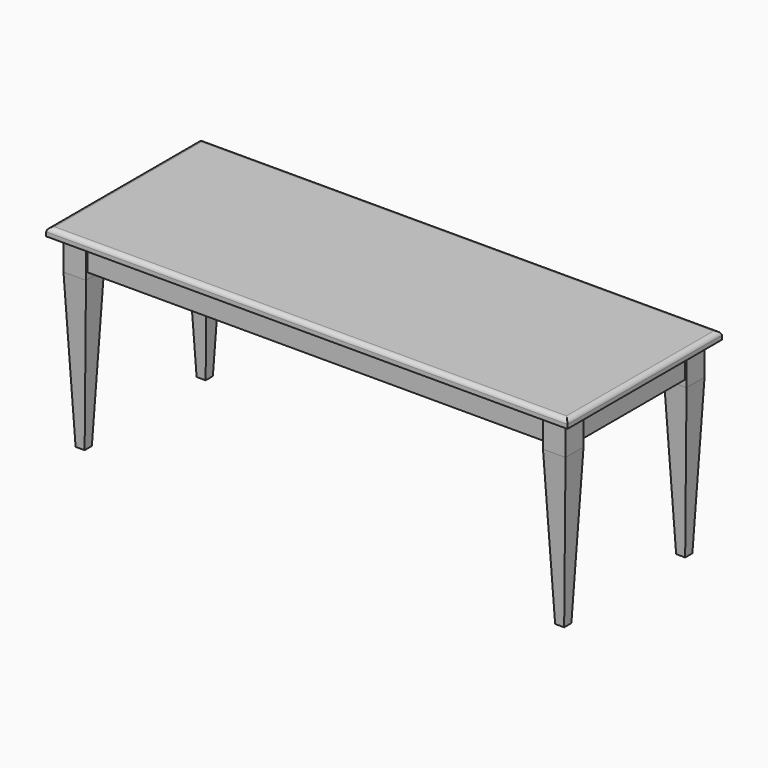
from build123d import *

# Parameters (mm, degrees)
F0_W        = 2057.4
F0_H        = 762
F1_DEPTH    = 15.875
F2_W        = 2057.4
F2_H        = 762
F3_DEPTH    = 15.875
F4_T1_DEPTH = 2151.3177665567
F4_T3_DEPTH = 855.9177665567
F6_W        = 88.9
F6_H        = 88.9
F7_DEPTH    = 127
F9_W        = 1968.5
F9_H        = 673.1
F10_DEPTH   = 101.6
F11_T       = -25.4
F12_W       = 88.9
F12_H       = 88.9
F13_DEPTH   = 609.6
F13_TAPER   = 2.5


# Not quite as in the source:
# - a fillet or chamfer that OpenCascade refuses, or shapes differently, is made with other operations: its cross-section is extruded or revolved along the edge and cut away or added


with BuildPart() as f1:
    # F0 (on Top) → F1 (new body)
    with BuildSketch(Plane.XY):
        Rectangle(F0_W, F0_H)
    extrude(amount=F1_DEPTH)

    # F6 (on face) → F7 (join)
    with BuildSketch(Plane(origin=(0, 0, 0), x_dir=(1, 0, 0), z_dir=(0, 0, -1))):
        with Locations((-946.15, 298.45)):
            Rectangle(F6_W, F6_H)
        with Locations((-946.15, -298.45)):
            Rectangle(F6_W, F6_H)
    extrude(amount=F7_DEPTH)

    # F8: F1 across plane


with BuildPart() as f3:
    # F2 (on face) → F3 (new body)
    with BuildSketch(Plane.XY.offset(15.875)):
        Rectangle(F2_W, F2_H)
    extrude(amount=F3_DEPTH)

    # F4: fillet of radius 19.05 on 4 edges, made by hand

    # F4_s2 → F4_t1 (cut)
    with BuildSketch(Plane.YZ.offset(-1075.6588832784)):
        with BuildLine():
            ThreePointArc((-381, 15.875), (-374.5131688129, 27.2496778315), (-362.2164466887, 31.75))
            Line((-362.2164466887, 31.75), (-381, 31.75))
            Line((-381, 31.75), (-381, 15.875))
        make_face()
        with BuildLine():
            ThreePointArc((381, 15.875), (374.5131688129, 27.2496778315), (362.2164466887, 31.75))
            Line((362.2164466887, 31.75), (381, 31.75))
            Line((381, 31.75), (381, 15.875))
        make_face()
    extrude(amount=F4_T1_DEPTH, mode=Mode.SUBTRACT)

    # F4_s4 → F4_t3 (cut)
    with BuildSketch(Plane.XZ.offset(-427.9588832784)):
        with BuildLine():
            ThreePointArc((-1028.7, 15.875), (-1022.2131688129, 27.2496778315), (-1009.9164466887, 31.75))
            Line((-1009.9164466887, 31.75), (-1028.7, 31.75))
            Line((-1028.7, 31.75), (-1028.7, 15.875))
        make_face()
        with BuildLine():
            ThreePointArc((1028.7, 15.875), (1022.2131688129, 27.2496778315), (1009.9164466887, 31.75))
            Line((1009.9164466887, 31.75), (1028.7, 31.75))
            Line((1028.7, 31.75), (1028.7, 15.875))
        make_face()
    extrude(amount=F4_T3_DEPTH, mode=Mode.SUBTRACT)


with BuildPart() as f1_1:
    add(f1.part)
    add(f1.part.mirror(Plane.YZ))

    # F12 (on face) → F13 (join)
    with BuildSketch(Plane(origin=(0, 0, -127), x_dir=(1, 0, 0), z_dir=(0, 0, -1))):
        with Locations((-946.15, 298.45)):
            Rectangle(F12_W, F12_H)
    extrude(amount=F13_DEPTH, taper=F13_TAPER)


with BuildPart() as f10:
    # F9 (on face) → F10 (new body)
    with BuildSketch(Plane(origin=(0, 0, 0), x_dir=(1, 0, 0), z_dir=(0, 0, -1))):
        Rectangle(F9_W, F9_H)
    extrude(amount=F10_DEPTH)

    # F11
    f11_openings = [f10.faces().sort_by_distance(p)[0] for p in [
        (0, 0, -101.6),
    ]]
    offset(amount=F11_T, openings=f11_openings)


with BuildPart() as f14_1:
    # F14: instance of F1
    add(f1_1.part.mirror(Plane.XZ))


with BuildPart() as f1_2:
    add(f1_1.part)

    add(f14_1.part)  # F15 merges F14_1
    # F15: F1, F14_1 across plane
    add(f1_1.part.mirror(Plane.YZ))
    add(f14_1.part.mirror(Plane.YZ))


solid = Compound([f3.part, f10.part, f1_2.part])
